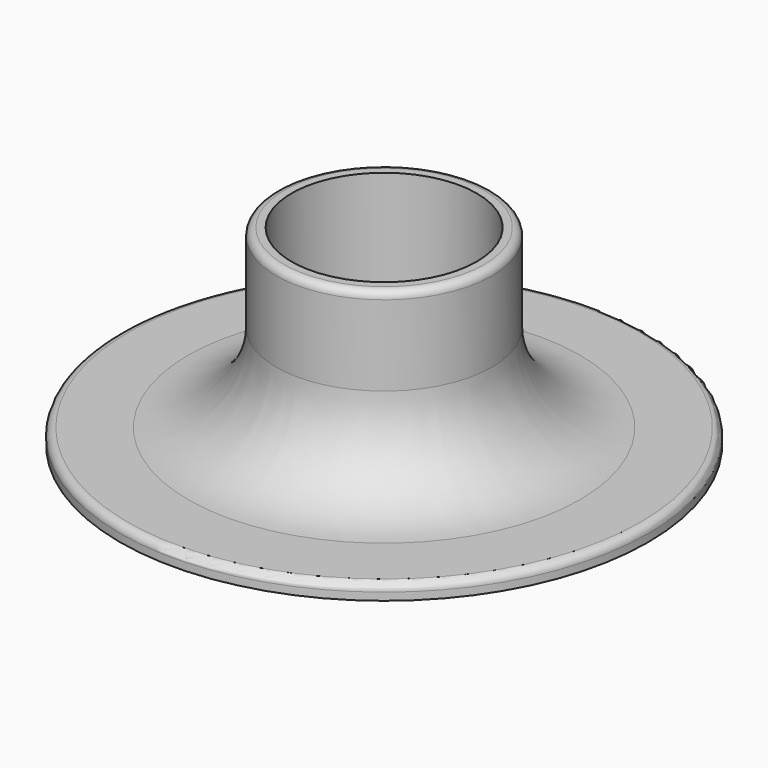
from build123d import *

# Parameters (mm, degrees)
F2_TEXT_SIZE = 11.3755189684
F3_DEPTH     = 0.5
F4_R         = 1


# Not quite as in the source:
# - Text() gives the source's letters only with a copy of the font that has no kerning and outlines rounded to 1/6400 em; it was checked with that copy


with BuildPart() as f1:
    # F0 (on Front) → F1 (revolve)
    with BuildSketch(Plane.XZ):
        with BuildLine():
            Line((0, 2), (0, 0))
            Line((0, 0), (34.65, 0))
            Line((34.65, 0), (34.65, 2))
            Line((34.65, 2), (25.7, 2))
            ThreePointArc((25.7, 2), (17.5329166773, 5.3829166773), (14.15, 13.55))
            Line((14.15, 13.55), (14.15, 25.1))
            Line((14.15, 25.1), (12.15, 25.1))
            Line((12.15, 25.1), (12.15, 2))
            Line((12.15, 2), (0, 2))
        make_face()
    revolve(axis=Axis((0, 0, 1), (0, 0, -1)))

    # F2 (on face) → F3 (cut)
    with BuildSketch(Plane.XY.offset(2)):
        with Locations((-9.224947542, -4.8280097544)):
            Text('3E8', F2_TEXT_SIZE, font='Open Sans', text_align=(TextAlign.LEFT, TextAlign.BOTTOM))
    extrude(amount=-F3_DEPTH, mode=Mode.SUBTRACT)

    # F4
    f4_edges = [f1.edges().sort_by_distance(p)[0] for p in [
        (-14.15, 0, 25.1),
        (-34.65, 0, 2),
    ]]
    fillet(f4_edges, radius=F4_R)


solid = f1.part
